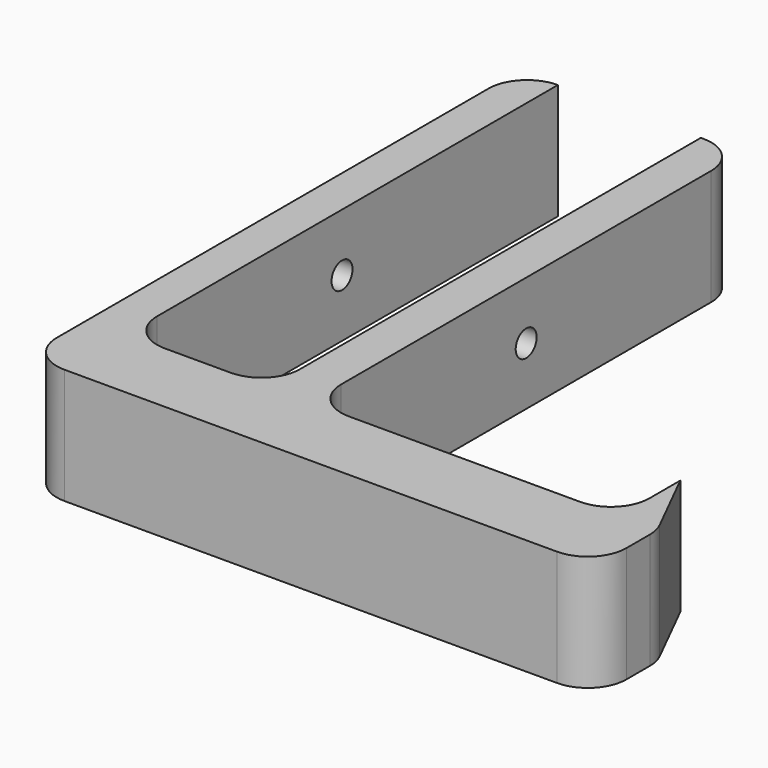
from build123d import *

# Parameters (mm, degrees)
F1_DEPTH = 15
F2_R     = 1.7
F3_DEPTH = 28.8924828911
F5_DEPTH = 1.38
F6_R     = 4.99999


# Not quite as in the source:
# - a fillet or chamfer is up to 0.001 mm smaller than in the source, because OpenCascade refuses the exact size


with BuildPart() as f1:
    # F0 (on Top) → F1 (new body)
    with BuildSketch(Plane.XY):
        Polygon((9.275, 35), (9.275, -35), (-9.275, -35), (-9.275, 35), (-14.275, 35), (-14.275, -35), (-14.275, -45), (59.6164828911, -45), (59.6164828911, -35), (54.6164828911, -25), (54.6164828911, -35), (14.6164828911, -35), (14.6164828911, 35), align=None)
    extrude(amount=F1_DEPTH)

    # F2 (on face) → F3 (cut, through all)
    with BuildSketch(Plane.YZ.offset(14.6164828911)):
        with Locations((0, 7.5)):
            Circle(F2_R)
    extrude(amount=-F3_DEPTH, mode=Mode.SUBTRACT)

    # F4 (on face) → F5 (cut)
    with BuildSketch(Plane(origin=(-14.275, 0, 0), x_dir=(0, -1, 0), z_dir=(-1, 0, 0))):
        Polygon((-2.2689865579, 3.57), (2.2689865579, 3.57), (4.5379731158, 7.5), (2.2689865579, 11.43), (-2.2689865579, 11.43), (-4.5379731158, 7.5), align=None)
    extrude(amount=-F5_DEPTH, mode=Mode.SUBTRACT)

    # F6 (radius 5 in the source; OpenCascade refuses exactly that, so slightly less here)
    f6_edges = [f1.edges().sort_by_distance(p)[0] for p in [
        (-9.275, -35, 7.5),
        (9.275, -35, 7.5),
        (-14.275, -45, 7.5),
        (59.616483, -45, 7.5),
        (54.616483, -35, 7.5),
        (14.616483, -35, 7.5),
        (59.616483, -35, 7.5),
        (14.616483, 35, 7.5),
        (-14.275, 35, 7.5),
    ]]
    fillet(f6_edges, radius=F6_R)


solid = f1.part
